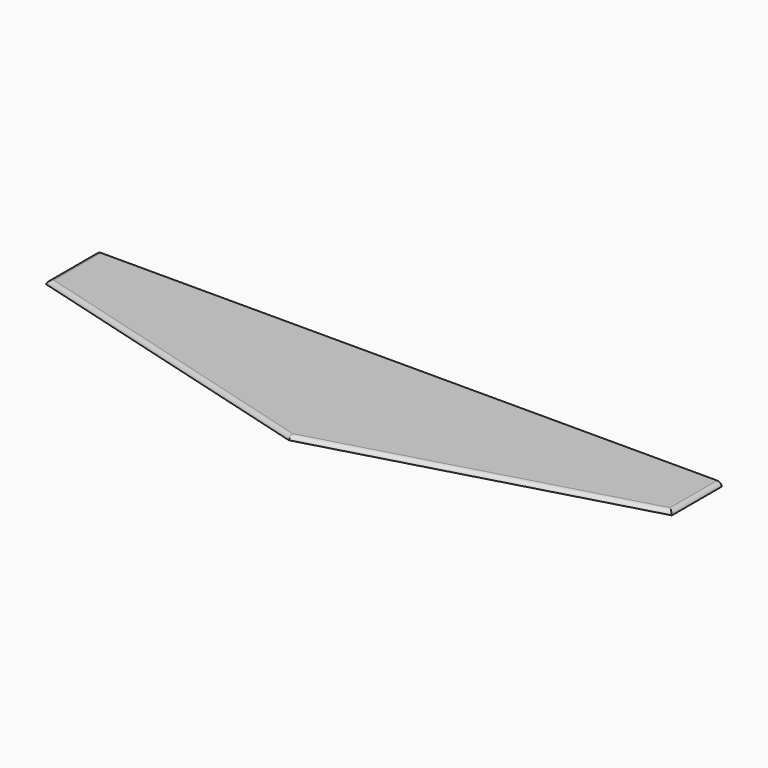
from build123d import *

# Parameters (mm, degrees)
F1_DEPTH    = 1.5
F2_T1_DEPTH = 69.364916731
F2_T3_DEPTH = 278.980016446
F2_T5_DEPTH = 278.980016446


# Not quite as in the source:
# - a fillet or chamfer that OpenCascade refuses, or shapes differently, is made with other operations: its cross-section is extruded or revolved along the edge and cut away or added


with BuildPart() as f1:
    # F0 (on Top) → F1 (new body, symmetric)
    with BuildSketch(Plane.XY):
        Polygon((-250, 10), (0, -60), (0, 60), (-250, 60), align=None)
        Polygon((0, 60), (0, -60), (250, 10), (250, 60), align=None)
    extrude(amount=F1_DEPTH, both=True)

    # F2: fillet of radius 4 on 4 edges, made by hand

    # F2_s2 → F2_t1 (cut)
    with BuildSketch(Plane.XZ.offset(-69.6824583655)):
        with BuildLine():
            ThreePointArc((250, -1.5), (248.5765063966, 0.6622776602), (246.1270166538, 1.5))
            Line((246.1270166538, 1.5), (250, 1.5))
            Line((250, 1.5), (250, -1.5))
        make_face()
        with BuildLine():
            ThreePointArc((-250, -1.5), (-248.5765063966, 0.6622776602), (-246.1270166538, 1.5))
            Line((-246.1270166538, 1.5), (-250, 1.5))
            Line((-250, 1.5), (-250, -1.5))
        make_face()
    extrude(amount=F2_T1_DEPTH, mode=Mode.SUBTRACT)

    # F2_s4 → F2_t3 (cut)
    with BuildSketch(Plane(origin=(-24.9024940432, -6.9726983321, 0), x_dir=(0, 0, 1), z_dir=(0.9629640197, 0.2696299255, 0))):
        with BuildLine():
            ThreePointArc((1.5, 53.9048578366), (0.6622776602, 56.3543475794), (-1.5, 57.7778411829))
            Line((-1.5, 57.7778411829), (1.5, 57.7778411829))
            Line((1.5, 57.7778411829), (1.5, 53.9048578366))
        make_face()
    extrude(amount=F2_T3_DEPTH, mode=Mode.SUBTRACT)

    # F2_s6 → F2_t5 (cut)
    with BuildSketch(Plane(origin=(-243.7452240135, 68.2486627238, 0), x_dir=(0, 0, 1), z_dir=(0.9629640197, -0.2696299255, 0))):
        with BuildLine():
            ThreePointArc((-1.5, 57.7778411829), (0.6622776602, 56.3543475794), (1.5, 53.9048578366))
            Line((1.5, 53.9048578366), (1.5, 57.7778411829))
            Line((1.5, 57.7778411829), (-1.5, 57.7778411829))
        make_face()
    extrude(amount=F2_T5_DEPTH, mode=Mode.SUBTRACT)


solid = f1.part
